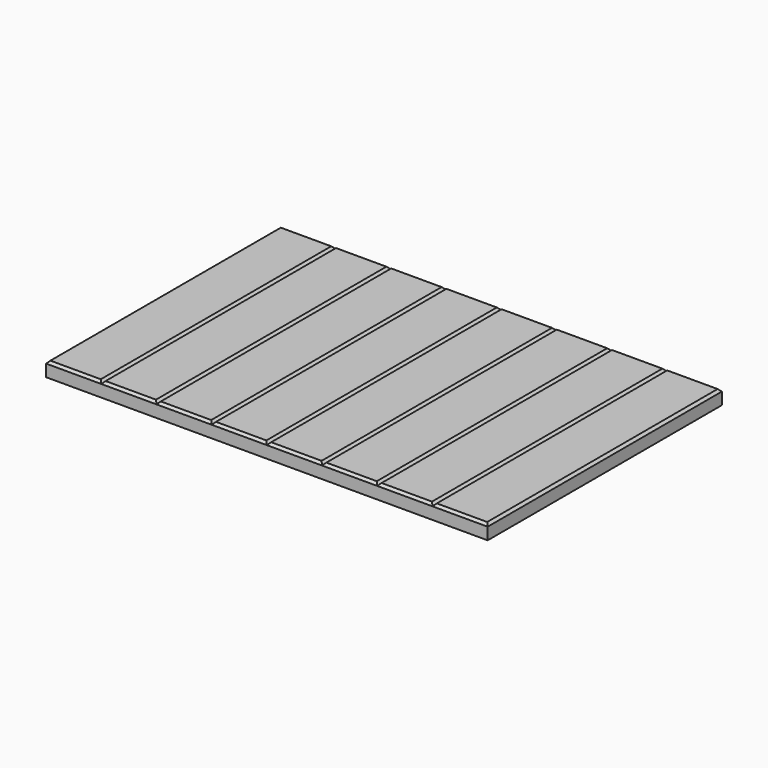
from build123d import *

# Parameters (mm, degrees)
F0_W     = 584.2
F0_H     = 387.35
F1_DEPTH = 19.05
F3_DEPTH = 387.351
F4_SIZE  = 3.17499


# Not quite as in the source:
# - a fillet or chamfer is up to 0.001 mm smaller than in the source, because OpenCascade refuses the exact size


with BuildPart() as f1:
    # F0 (on Top) → F1 (new body)
    with BuildSketch(Plane.XY):
        Rectangle(F0_W, F0_H)
    extrude(amount=F1_DEPTH)

    # F2 (on face) → F3 (cut, through all)
    with BuildSketch(Plane.XZ.offset(193.675)):
        Polygon((-219.075, 19.05), (-222.25, 19.05), (-219.075, 15.875), (-215.9, 19.05), align=None)
        Polygon((-146.05, 19.05), (-149.225, 19.05), (-146.05, 15.875), (-142.875, 19.05), align=None)
        Polygon((-73.025, 19.05), (-76.2, 19.05), (-73.025, 15.875), (-69.85, 19.05), align=None)
        Polygon((0, 19.05), (-3.175, 19.05), (0, 15.875), (3.175, 19.05), align=None)
        Polygon((73.025, 19.05), (69.85, 19.05), (73.025, 15.875), (76.2, 19.05), align=None)
        Polygon((146.05, 19.05), (142.875, 19.05), (146.05, 15.875), (149.225, 19.05), align=None)
        Polygon((219.075, 19.05), (215.9, 19.05), (219.075, 15.875), (222.25, 19.05), align=None)
    extrude(amount=-F3_DEPTH, mode=Mode.SUBTRACT)

    # F4 (size 3.175 in the source; OpenCascade refuses exactly that, so slightly less here)
    f4_edges = [f1.edges().sort_by_distance(p)[0] for p in [
        (-292.1, 0, 19.05),
        (-257.175, -193.675, 19.05),
        (-182.5625, -193.675, 19.05),
        (-109.5375, -193.675, 19.05),
        (-36.5125, -193.675, 19.05),
        (36.5125, -193.675, 19.05),
        (109.5375, -193.675, 19.05),
        (182.5625, -193.675, 19.05),
        (257.175, -193.675, 19.05),
        (257.175, 193.675, 19.05),
        (182.5625, 193.675, 19.05),
        (109.5375, 193.675, 19.05),
        (36.5125, 193.675, 19.05),
        (-36.5125, 193.675, 19.05),
        (-109.5375, 193.675, 19.05),
        (-182.5625, 193.675, 19.05),
        (-257.175, 193.675, 19.05),
        (292.1, 0, 19.05),
    ]]
    chamfer(f4_edges, length=F4_SIZE)


solid = f1.part
